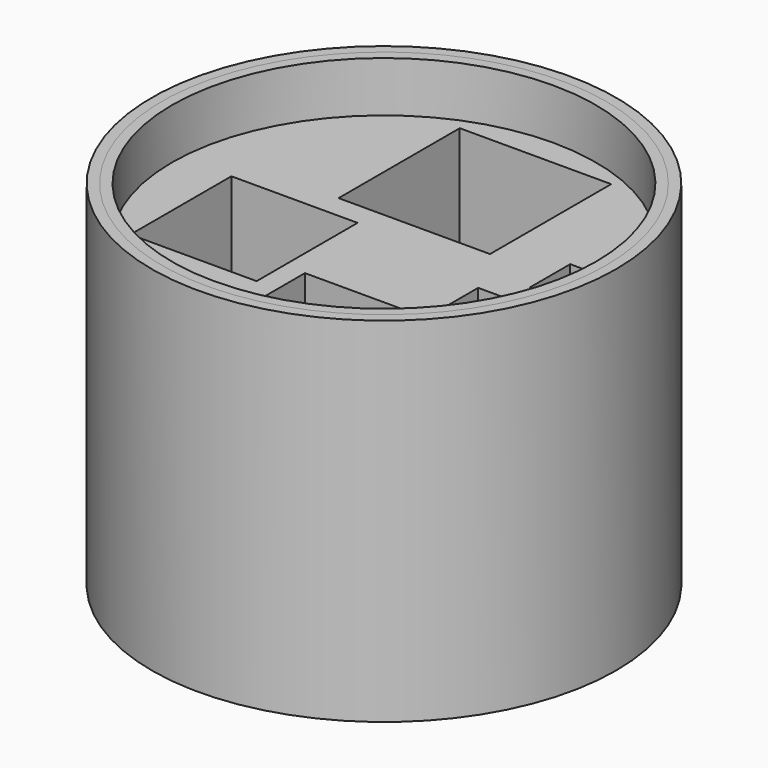
from build123d import *

# Parameters (mm, degrees)
F0_R     = 26.67
F0_W     = 15.875
F0_H     = 15.875
F0_W_2   = 12.7
F0_H_2   = 12.7
F0_W_3   = 9.525
F0_H_3   = 9.525
F0_W_4   = 19.05
F0_H_4   = 19.05
F0_W_5   = 6.35
F0_H_5   = 6.35
F1_DEPTH = 2.54
F0_R_2   = 27.94
F2_DEPTH = 44.45
F0_R_3   = 29.21
F3_DEPTH = 38.1
F4_DEPTH = 2.54
F5_DEPTH = 38.1
F6_DEPTH = 44.45


with BuildPart() as f1:
    # F0 (on Top) → F1 (new body)
    with BuildSketch(Plane.XY):
        Circle(F0_R)
        with Locations((-12.3339120969, -6.5917588277)):
            Rectangle(F0_W, F0_H, mode=Mode.SUBTRACT)
        with Locations((4.5904321199, -16.5795920581)):
            Rectangle(F0_W_2, F0_H_2, mode=Mode.SUBTRACT)
        with Locations((18.2479810312, -6.8110866129)):
            Rectangle(F0_W_3, F0_H_3, mode=Mode.SUBTRACT)
        with Locations((0.3825599574, 13.8187071994)):
            Rectangle(F0_W_4, F0_H_4, mode=Mode.SUBTRACT)
        with Locations((20.5775478005, 4.3574731482)):
            Rectangle(F0_W_5, F0_H_5, mode=Mode.SUBTRACT)
        with Locations((0.3825599574, 13.8187071994)):
            Rectangle(F0_W_4, F0_H_4)
        with Locations((-12.3339120969, -6.5917588277)):
            Rectangle(F0_W, F0_H)
        with Locations((4.5904321199, -16.5795920581)):
            Rectangle(F0_W_2, F0_H_2)
        with Locations((18.2479810312, -6.8110866129)):
            Rectangle(F0_W_3, F0_H_3)
        with Locations((20.5775478005, 4.3574731482)):
            Rectangle(F0_W_5, F0_H_5)
    extrude(amount=F1_DEPTH)

    # F0 (on Top) → F2 (join)
    with BuildSketch(Plane.XY):
        Circle(F0_R_2)
        Circle(F0_R, mode=Mode.SUBTRACT)
    extrude(amount=F2_DEPTH)

    # F0 (on Top) → F3 (join)
    with BuildSketch(Plane.XY):
        Circle(F0_R_3)
        Circle(F0_R_2, mode=Mode.SUBTRACT)
        Circle(F0_R)
        with Locations((-12.3339120969, -6.5917588277)):
            Rectangle(F0_W, F0_H, mode=Mode.SUBTRACT)
        with Locations((4.5904321199, -16.5795920581)):
            Rectangle(F0_W_2, F0_H_2, mode=Mode.SUBTRACT)
        with Locations((18.2479810312, -6.8110866129)):
            Rectangle(F0_W_3, F0_H_3, mode=Mode.SUBTRACT)
        with Locations((0.3825599574, 13.8187071994)):
            Rectangle(F0_W_4, F0_H_4, mode=Mode.SUBTRACT)
        with Locations((20.5775478005, 4.3574731482)):
            Rectangle(F0_W_5, F0_H_5, mode=Mode.SUBTRACT)
    extrude(amount=F3_DEPTH)


with BuildPart() as f4:
    # F0 (on Top) → F4 (new body)
    with BuildSketch(Plane.XY):
        Circle(F0_R)
        with Locations((-12.3339120969, -6.5917588277)):
            Rectangle(F0_W, F0_H, mode=Mode.SUBTRACT)
        with Locations((4.5904321199, -16.5795920581)):
            Rectangle(F0_W_2, F0_H_2, mode=Mode.SUBTRACT)
        with Locations((18.2479810312, -6.8110866129)):
            Rectangle(F0_W_3, F0_H_3, mode=Mode.SUBTRACT)
        with Locations((0.3825599574, 13.8187071994)):
            Rectangle(F0_W_4, F0_H_4, mode=Mode.SUBTRACT)
        with Locations((20.5775478005, 4.3574731482)):
            Rectangle(F0_W_5, F0_H_5, mode=Mode.SUBTRACT)
        with Locations((-12.3339120969, -6.5917588277)):
            Rectangle(F0_W, F0_H)
        with Locations((4.5904321199, -16.5795920581)):
            Rectangle(F0_W_2, F0_H_2)
        with Locations((18.2479810312, -6.8110866129)):
            Rectangle(F0_W_3, F0_H_3)
        with Locations((20.5775478005, 4.3574731482)):
            Rectangle(F0_W_5, F0_H_5)
        with Locations((0.3825599574, 13.8187071994)):
            Rectangle(F0_W_4, F0_H_4)
    extrude(amount=F4_DEPTH)

    # F0 (on Top) → F5 (join)
    with BuildSketch(Plane.XY):
        Circle(F0_R_2)
        Circle(F0_R, mode=Mode.SUBTRACT)
    extrude(amount=F5_DEPTH)

    # F0 (on Top) → F6 (join)
    with BuildSketch(Plane.XY):
        Circle(F0_R_3)
        Circle(F0_R_2, mode=Mode.SUBTRACT)
    extrude(amount=F6_DEPTH)


solid = Compound([f1.part, f4.part])
